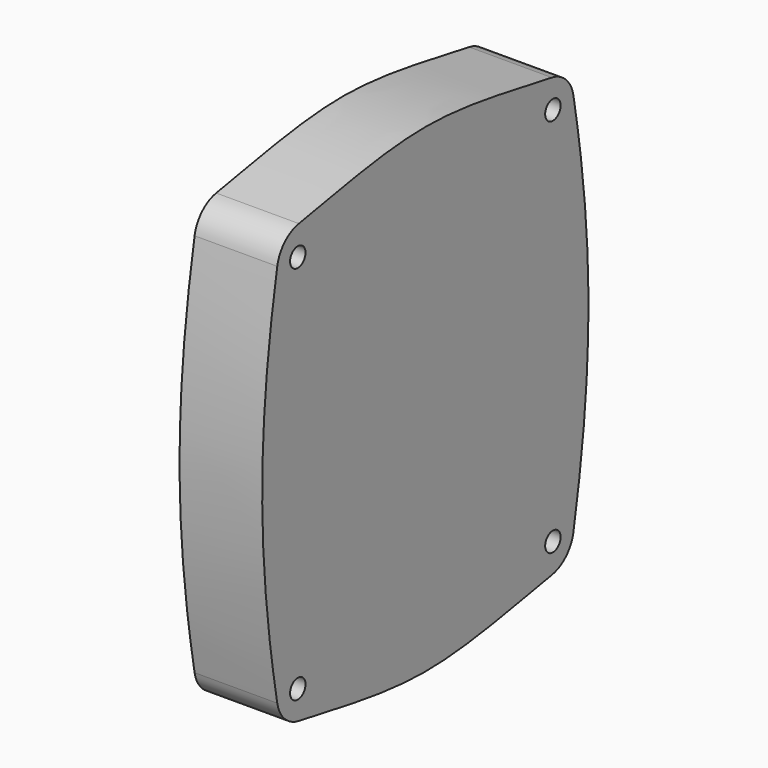
from build123d import *

# Parameters (mm, degrees)
F0_R     = 3
F0_R_2   = 1.75
F1_DEPTH = 15


with BuildPart() as f1:
    # F0 (on Right) → F1 (new body)
    with BuildSketch(Plane.YZ):
        with BuildLine():
            ThreePointArc((33.6642538877, 94.2964592226), (31.9768261624, 97.4851943073), (28.7658063512, 99.1298205687))
            add(Edge.make_bspline(
                [(28.7658063512, 99.1298205687), (19.203840359, 100.7513284104), (0.0799083746, 105.0635755317), (-19.0440236097, 100.7513284104), (-28.6059896019, 99.1298205687)],
                knots=[0.0624771081, 0.0624771081, 0.0624771081, 0.0624771081, 0.5, 0.9375228919, 0.9375228919, 0.9375228919, 0.9375228919], degree=3))
            ThreePointArc((-28.6059896019, 99.1298205687), (-31.8170094131, 97.4851943073), (-33.5044371384, 94.2964592226))
            add(Edge.make_bspline(
                [(-33.5044371384, 94.2964592226), (-35.6369863321, 82.6667901388), (-38.2031969186, 59.4074519711), (-35.6369863321, 36.1481138033), (-33.5044371384, 24.5184447195)],
                knots=[0.0534866237, 0.0534866237, 0.0534866237, 0.0534866237, 0.5, 0.9465133763, 0.9465133763, 0.9465133763, 0.9465133763], degree=3))
            ThreePointArc((-33.5044371384, 24.5184447195), (-31.8170094131, 21.3297096348), (-28.6059896019, 19.6850833734))
            add(Edge.make_bspline(
                [(-28.6059896019, 19.6850833734), (-19.0440236097, 18.0635755317), (0.0799083746, 13.7513284104), (19.203840359, 18.0635755317), (28.7658063512, 19.6850833734)],
                knots=[0.0624771081, 0.0624771081, 0.0624771081, 0.0624771081, 0.5, 0.9375228919, 0.9375228919, 0.9375228919, 0.9375228919], degree=3))
            ThreePointArc((28.7658063512, 19.6850833734), (31.9768261624, 21.3297096348), (33.6642538877, 24.5184447195))
            add(Edge.make_bspline(
                [(33.6642538877, 24.5184447195), (35.7968030814, 36.1481138033), (38.3630136679, 59.4074519711), (35.7968030814, 82.6667901388), (33.6642538877, 94.2964592226)],
                knots=[0.0534866237, 0.0534866237, 0.0534866237, 0.0534866237, 0.5, 0.9465133763, 0.9465133763, 0.9465133763, 0.9465133763], degree=3))
        make_face()
        with Locations((-28.8455340613, 24.9354520307)):
            Circle(F0_R, mode=Mode.SUBTRACT)
        with Locations((29.0053508105, 24.9354520307)):
            Circle(F0_R, mode=Mode.SUBTRACT)
        with Locations((-28.8455340613, 93.8794519114)):
            Circle(F0_R, mode=Mode.SUBTRACT)
        with Locations((29.0053508105, 93.8794519114)):
            Circle(F0_R, mode=Mode.SUBTRACT)
        with Locations((29.0053508105, 93.8794519114)):
            Circle(F0_R)
        with Locations((29.0053508105, 93.8794519114)):
            Circle(F0_R_2, mode=Mode.SUBTRACT)
        with Locations((-28.8455340613, 93.8794519114)):
            Circle(F0_R)
        with Locations((-28.8455340613, 93.8794519114)):
            Circle(F0_R_2, mode=Mode.SUBTRACT)
        with Locations((-28.8455340613, 24.9354520307)):
            Circle(F0_R)
        with Locations((-28.8455340613, 24.9354520307)):
            Circle(F0_R_2, mode=Mode.SUBTRACT)
        with Locations((29.0053508105, 24.9354520307)):
            Circle(F0_R)
        with Locations((29.0053508105, 24.9354520307)):
            Circle(F0_R_2, mode=Mode.SUBTRACT)
    extrude(amount=F1_DEPTH)


solid = f1.part
